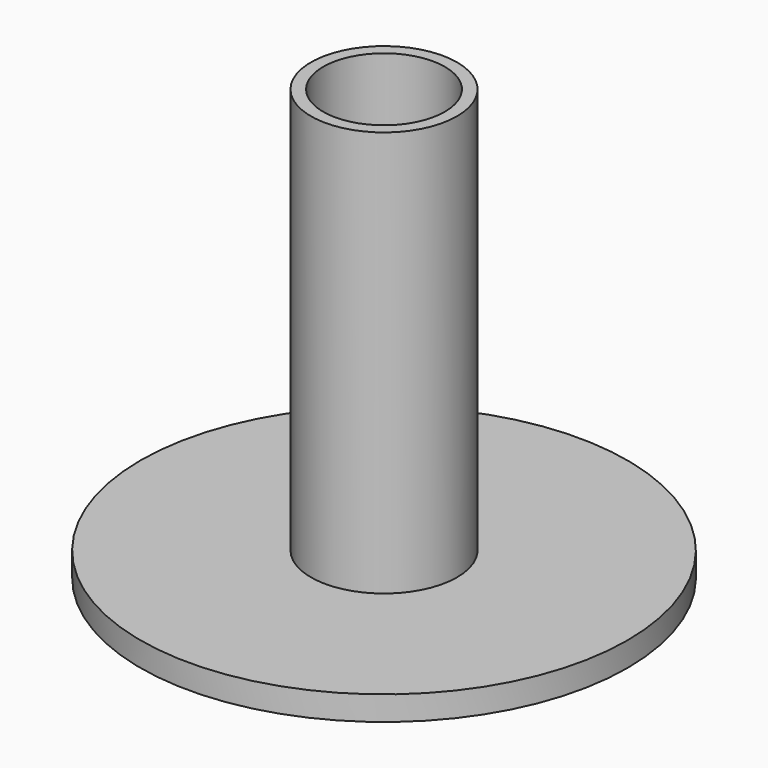
from build123d import *

# Parameters (mm, degrees)
F0_R     = 30
F1_DEPTH = 3
F2_R     = 9
F3_DEPTH = 50
F4_T     = 1.5


# Not quite as in the source:
# - a shell that OpenCascade refuses in one call is made with other operations: the cavity is built on its own and cut out


with BuildPart() as f1:
    # F0 (on Top) → F1 (new body)
    with BuildSketch(Plane.XY):
        Circle(F0_R)
    extrude(amount=F1_DEPTH)

    # F2 (on face) → F3 (join)
    with BuildSketch(Plane.XY.offset(3)):
        Circle(F2_R)
    extrude(amount=F3_DEPTH)

    # F4: shell of thickness 1.5, made by hand


with BuildPart() as f4_core1:
    # F4_t2: copy of F1
    add(f1.part)

    # the walls: a layer under each face that stays
    f4_faces = [f4_core1.faces().sort_by_distance(p)[0] for p in [
        (-30, 0, 1.5),
        (0, 0, 0),
        (-20, -20, 3),
        (-9, 0, 28),
    ]]
    thicken(f4_faces, amount=-F4_T, mode=Mode.SUBTRACT)

    # F4_s3 → F4_t4 (revolve, cut)
    with BuildSketch(Plane.XZ):
        Polygon((9.015, 3.015), (9, 1.5), (7.5, 1.5), (7.5, 3), align=None)
    revolve(axis=Axis((0, 0, 3), (0, 0, 1)), mode=Mode.SUBTRACT)


with BuildPart() as f1_1:
    add(f1.part)

    # what is left inside the walls is the cavity
    f4_cavity = [f4_core1.part.solids().sort_by_distance(p)[0] for p in [
        (-7.485, 0, 18.666667),
    ]]
    add(f4_cavity, mode=Mode.SUBTRACT)


solid = f1_1.part
